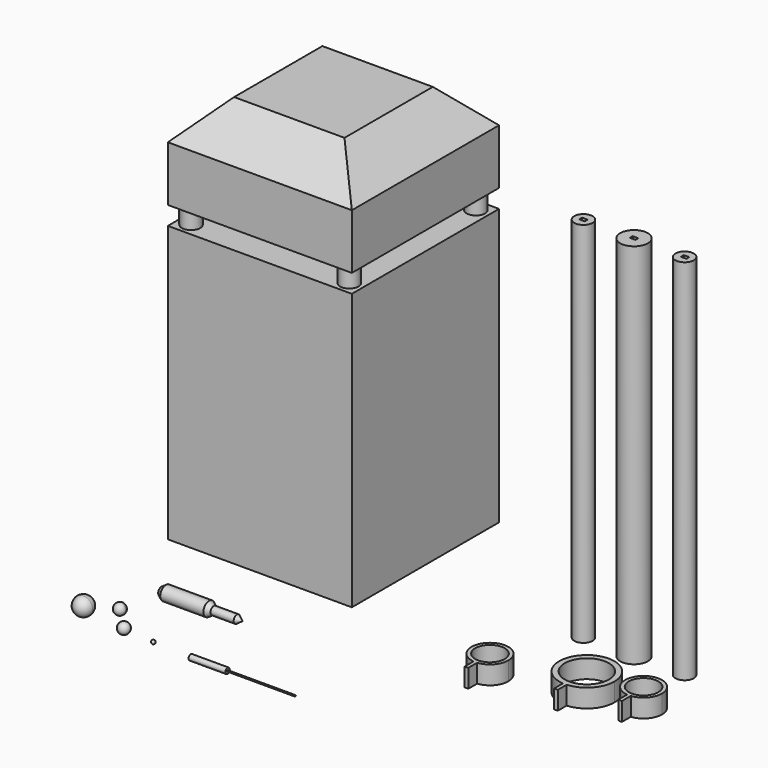
from build123d import *

# Parameters (mm, degrees)
F0_W      = 50
F0_H      = 50
F1_DEPTH  = 75
F2_R      = 2.5
F3_DEPTH  = 5
F4_W      = 50
F4_H      = 50
F4_R      = 2.5
F5_DEPTH  = 25
F6_SIZE   = 10
F7_R      = 2.5
F8_DEPTH  = 100
F7_R_2    = 3.75
F10_W     = 1.5
F10_H     = 1
F11_DEPTH = 35
F13_W     = 1.5
F13_H     = 1
F14_DEPTH = 35
F12_W     = 1.5
F12_H     = 1
F15_DEPTH = 35
F9_R      = 4
F16_DEPTH = 5
F9_R_2    = 6
F27_W     = 18.4128382243
F27_H     = 0.1725424081
F29_R     = 0.75
F29_R_2   = 0.1725424081
F30_DEPTH = 10


with BuildPart() as f1:
    # F0 (on Top) → F1 (new body)
    with BuildSketch(Plane.XY):
        with Locations((-47.1544858068, 46.3805288076)):
            Rectangle(F0_W, F0_H)
    extrude(amount=F1_DEPTH)

    # F2 (on face) → F3 (join)
    with BuildSketch(Plane.XY.offset(75)):
        with Locations((-68.6544858068, 67.8805288076)):
            Circle(F2_R)
        with Locations((-25.6544858068, 67.8805288076)):
            Circle(F2_R)
        with Locations((-68.6544858068, 24.8805288076)):
            Circle(F2_R)
        with Locations((-25.6544858068, 24.8805288076)):
            Circle(F2_R)
    extrude(amount=F3_DEPTH)

    # F4 (on face) → F5 (join)
    with BuildSketch(Plane.XY.offset(80)):
        with Locations((-47.1544858068, 46.3805288076)):
            Rectangle(F4_W, F4_H)
        with Locations((-68.6544858068, 24.8805288076)):
            Circle(F4_R, mode=Mode.SUBTRACT)
        with Locations((-68.6544858068, 24.8805288076)):
            Circle(F4_R)
    extrude(amount=F5_DEPTH)

    # F6
    f6_edges = [f1.edges().sort_by_distance(p)[0] for p in [
        (-47.154486, 21.380529, 105),
        (-22.154486, 46.380529, 105),
        (-47.154486, 71.380529, 105),
        (-72.154486, 46.380529, 105),
    ]]
    chamfer(f6_edges, length=F6_SIZE)


with BuildPart() as f8:
    # F7 (on Top) → F8 (new body)
    with BuildSketch(Plane.XY):
        with Locations((24.8829479516, 41.2498153746)):
            Circle(F7_R)
    extrude(amount=F8_DEPTH)

    # F13 (on face) → F14 (cut)
    with BuildSketch(Plane.XY.offset(100)):
        with Locations((24.8809913173, 41.2483455206)):
            Rectangle(F13_W, F13_H)
    extrude(amount=-F14_DEPTH, mode=Mode.SUBTRACT)


with BuildPart() as f8b:
    # F7 (on Top) → F8, piece 2 (new body)
    with BuildSketch(Plane.XY):
        with Locations((38.6329479516, 41.2498153746)):
            Circle(F7_R_2)
    extrude(amount=F8_DEPTH)

    # F12 (on face) → F15 (cut)
    with BuildSketch(Plane.XY.offset(100)):
        with Locations((38.594292134, 41.3151393533)):
            Rectangle(F12_W, F12_H)
    extrude(amount=-F15_DEPTH, mode=Mode.SUBTRACT)


with BuildPart() as f8c:
    # F7 (on Top) → F8, piece 3 (new body)
    with BuildSketch(Plane.XY):
        with Locations((52.3829479516, 41.2498153746)):
            Circle(F7_R)
    extrude(amount=F8_DEPTH)

    # F10 (on face) → F11 (cut)
    with BuildSketch(Plane.XY.offset(100)):
        with Locations((52.4813026488, 41.281630367)):
            Rectangle(F10_W, F10_H)
        with Locations((38.6107728183, 41.281630367)):
            Rectangle(F10_W, F10_H)
        with Locations((24.78091757, 41.3629795313)):
            Rectangle(F10_W, F10_H)
    extrude(amount=-F11_DEPTH, mode=Mode.SUBTRACT)


with BuildPart() as f16:
    # F9 (on Top) → F16 (new body)
    with BuildSketch(Plane.XY):
        with BuildLine():
            ThreePointArc((20.5274762363, 10.6018343975), (20.0274762363, 10.576771583), (19.5274762363, 10.6018343975))
            Line((19.5274762363, 10.6018343975), (19.5274762363, 7.6018343975))
            Line((19.5274762363, 7.6018343975), (20.5274762363, 7.6018343975))
            Line((20.5274762363, 7.6018343975), (20.5274762363, 10.6018343975))
        make_face()
        with BuildLine():
            ThreePointArc((20.5274762363, 10.6018343975), (23.7355754798, 12.2226696168), (25.0274762363, 15.576771583))
            ThreePointArc((25.0274762363, 15.576771583), (16.67337427, 19.2848708266), (19.5274762363, 10.6018343975))
            ThreePointArc((19.5274762363, 10.6018343975), (20.0274762363, 10.576771583), (20.5274762363, 10.6018343975))
        make_face()
        with Locations((20.0274762363, 15.576771583)):
            Circle(F9_R, mode=Mode.SUBTRACT)
    extrude(amount=F16_DEPTH)


with BuildPart() as f16b:
    # F9 (on Top) → F16, piece 2 (new body)
    with BuildSketch(Plane.XY):
        with BuildLine():
            ThreePointArc((41.6674405202, 14.576771583), (41.1674405202, 14.5600863566), (40.6674405202, 14.576771583))
            Line((40.6674405202, 14.576771583), (40.6674405202, 11.576771583))
            Line((40.6674405202, 11.576771583), (41.6674405202, 11.576771583))
            Line((41.6674405202, 11.576771583), (41.6674405202, 14.576771583))
        make_face()
        with BuildLine():
            ThreePointArc((41.6674405202, 14.576771583), (46.6446660952, 16.9366109736), (48.6674405202, 22.0600863566))
            ThreePointArc((48.6674405202, 22.0600863566), (36.0439651372, 27.5373119316), (40.6674405202, 14.576771583))
            ThreePointArc((40.6674405202, 14.576771583), (41.1674405202, 14.5600863566), (41.6674405202, 14.576771583))
        make_face()
        with Locations((41.1674405202, 22.0600863566)):
            Circle(F9_R_2, mode=Mode.SUBTRACT)
    extrude(amount=F16_DEPTH)


with BuildPart() as f16c:
    # F9 (on Top) → F16, piece 3 (new body)
    with BuildSketch(Plane.XY):
        with BuildLine():
            ThreePointArc((55.5025293472, 19.0600863566), (55.0025293472, 19.0350235421), (54.5025293472, 19.0600863566))
            Line((54.5025293472, 19.0600863566), (54.5025293472, 16.0600863566))
            Line((54.5025293472, 16.0600863566), (55.5025293472, 16.0600863566))
            Line((55.5025293472, 16.0600863566), (55.5025293472, 19.0600863566))
        make_face()
        with BuildLine():
            ThreePointArc((55.5025293472, 19.0600863566), (58.7106285907, 20.6809215759), (60.0025293472, 24.0350235421))
            ThreePointArc((60.0025293472, 24.0350235421), (51.6484273809, 27.7431227857), (54.5025293472, 19.0600863566))
            ThreePointArc((54.5025293472, 19.0600863566), (55.0025293472, 19.0350235421), (55.5025293472, 19.0600863566))
        make_face()
        with Locations((55.0025293472, 24.0350235421)):
            Circle(F9_R, mode=Mode.SUBTRACT)
    extrude(amount=F16_DEPTH)


with BuildPart() as f21:
    # F17 (on Top) → F21 (revolve)
    with BuildSketch(Plane.XY):
        with BuildLine():
            ThreePointArc((-66.8653695327, -16.1144445679), (-65.2487937151, -15.3092323136), (-64.5964568853, -13.6251477525))
            ThreePointArc((-64.5964568853, -13.6251477525), (-65.4123723242, -11.7774845822), (-67.327544238, -11.135850937))
            Line((-67.327544238, -11.135850937), (-66.8653695327, -16.1144445679))
        make_face()
    revolve(axis=Axis((-67.0964568853, -13.6251477525, 0), (-0.0924349411, 0.9957187262, 0)))


with BuildPart() as f22:
    # F18 (on Top) → F22 (revolve)
    with BuildSketch(Plane.XY):
        with BuildLine():
            ThreePointArc((-60.6423460645, -11.332890958), (-59.2856783207, -11.1326644557), (-58.658798981, -9.9129676439))
            ThreePointArc((-58.658798981, -9.9129676439), (-58.9391021692, -9.0398469836), (-59.6752518974, -8.4930443298))
            Line((-59.6752518974, -8.4930443298), (-60.6423460645, -11.332890958))
        make_face()
    revolve(axis=Axis((-60.158798981, -9.9129676439, 0), (0.3223647224, 0.9466155427, 0)))


with BuildPart() as f23:
    # F19 (on Top) → F23 (revolve)
    with BuildSketch(Plane.XY):
        with BuildLine():
            Line((-54.8395033445, -17.5165602354), (-53.1109123013, -15.0646277312))
            ThreePointArc((-53.1109123013, -15.0646277312), (-55.201174075, -15.4262984617), (-54.8395033445, -17.5165602354))
        make_face()
    revolve(axis=Axis((-53.9752078229, -16.2905939833, 0), (-0.5761970144, -0.8173108347, 0)))


with BuildPart() as f24:
    # F20 (on Top) → F24 (revolve)
    with BuildSketch(Plane.XY):
        with BuildLine():
            Line((-45.1707579334, -17.86929287), (-45.0367656187, -16.878310499))
            ThreePointArc((-45.0367656187, -16.878310499), (-45.5992529615, -17.3068055272), (-45.1707579334, -17.86929287))
        make_face()
    revolve(axis=Axis((-45.103761776, -17.3738016845, 0), (-0.1339923147, -0.990982371, 0)))


with BuildPart() as f26:
    # F25 (on Top) → F26 (revolve)
    with BuildSketch(Plane.XY):
        Polygon((-57.1240112185, 3.8274246035), (-58.3320297301, 3.0066801119), (-58.3320297301, 1.9137123018), (-36.2616623452, 1.9137123018), (-37.8148290029, 3.0066801119), (-44.1159155295, 3.0066801119), (-45.3889928758, 3.8274246035), align=None)
    revolve(axis=Axis((-47.2968460376, 1.9137123018, 0), (-1, 0, 0)))


with BuildPart() as f28:
    # F27 (on Top) → F28 (revolve)
    with BuildSketch(Plane.XY):
        with Locations((-15.3013214003, -17.8114576265)):
            Rectangle(F27_W, F27_H)
    revolve(axis=Axis((-15.3013214003, -17.8977288306, 0), (1, 0, 0)))

    # F29 (on face) → F30 (join)
    with BuildSketch(Plane(origin=(-24.5077405125, 0, 0), x_dir=(0, -1, 0), z_dir=(-1, 0, 0))):
        with Locations((17.8977288306, 0)):
            Circle(F29_R)
        with Locations((17.8977288306, 0)):
            Circle(F29_R_2, mode=Mode.SUBTRACT)
        with Locations((17.8977288306, 0)):
            Circle(F29_R_2)
    extrude(amount=F30_DEPTH)


solid = Compound([f1.part, f8.part, f8b.part, f8c.part, f16.part, f16b.part, f16c.part, f21.part, f22.part, f23.part, f24.part, f26.part, f28.part])
